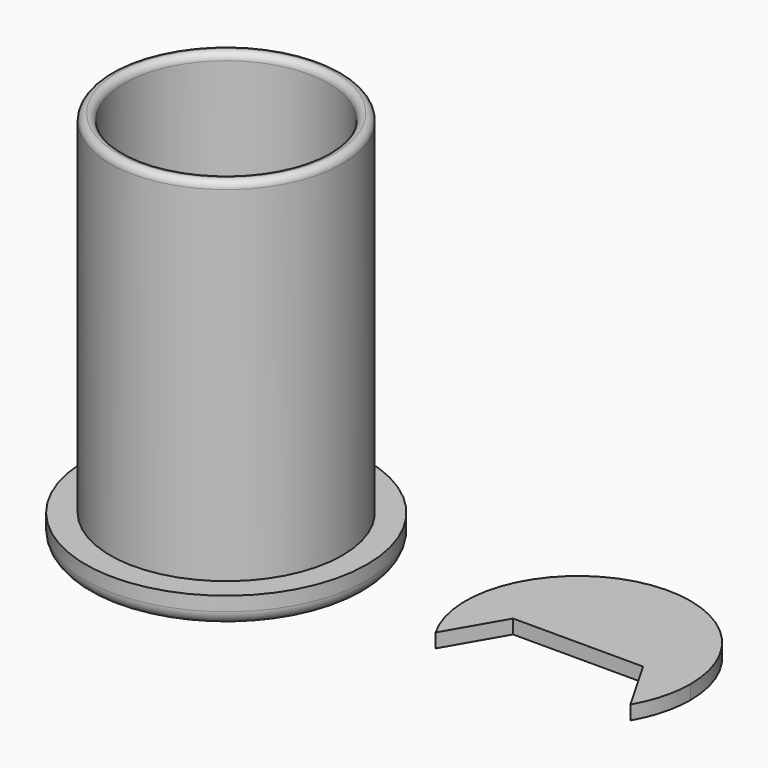
from build123d import *

# Parameters (mm, degrees)
F0_R          = 16.5
F0_R_2        = 14.5
F1_DEPTH      = 52
F0_R_3        = 20
F2_DEPTH      = 2
F2_DEPTH_BACK = 2
F3_R          = 1.99999
F4_R          = 0.99999
F5_DEPTH      = 2
F6_R          = 0.5


# Not quite as in the source:
# - a fillet or chamfer is up to 0.001 mm smaller than in the source, because OpenCascade refuses the exact size


with BuildPart() as f1:
    # F0 (on Top) → F1 (new body)
    with BuildSketch(Plane.XY):
        Circle(F0_R)
        Circle(F0_R_2, mode=Mode.SUBTRACT)
    extrude(amount=F1_DEPTH)

    # F0 (on Top) → F2 (join, two sides)
    with BuildSketch(Plane.XY) as f2_sk:
        Circle(F0_R_3)
        Circle(F0_R, mode=Mode.SUBTRACT)
    extrude(amount=F2_DEPTH)
    extrude(f2_sk.sketch, amount=-F2_DEPTH_BACK)

    # F3 (radius 2 in the source; OpenCascade refuses exactly that, so slightly less here)
    f3_edges = [f1.edges().sort_by_distance(p)[0] for p in [
        (-20, 0, -2),
    ]]
    fillet(f3_edges, radius=F3_R)

    # F4 (radius 1 in the source; OpenCascade refuses exactly that, so slightly less here)
    f4_edges = [f1.edges().sort_by_distance(p)[0] for p in [
        (-16.5, 0, 52),
        (-14.5, 0, 52),
    ]]
    fillet(f4_edges, radius=F4_R)

    # F6
    f6_edges = [f1.edges().sort_by_distance(p)[0] for p in [
        (-14.5, 0, 0),
    ]]
    fillet(f6_edges, radius=F6_R)


with BuildPart() as f5:
    # F0 (on Top) → F5 (new body)
    with BuildSketch(Plane.XY):
        with BuildLine():
            ThreePointArc((63.8564064606, -8), (65.4548132206, -4.1411047216), (66, 0))
            ThreePointArc((66, 0), (45.8588952784, 15.4548132206), (36.1435935394, -8))
            Line((36.1435935394, -8), (40.762395693, 0))
            Line((40.762395693, 0), (59.237604307, 0))
            Line((59.237604307, 0), (63.8564064606, -8))
        make_face()
    extrude(amount=F5_DEPTH)


solid = Compound([f1.part, f5.part])
